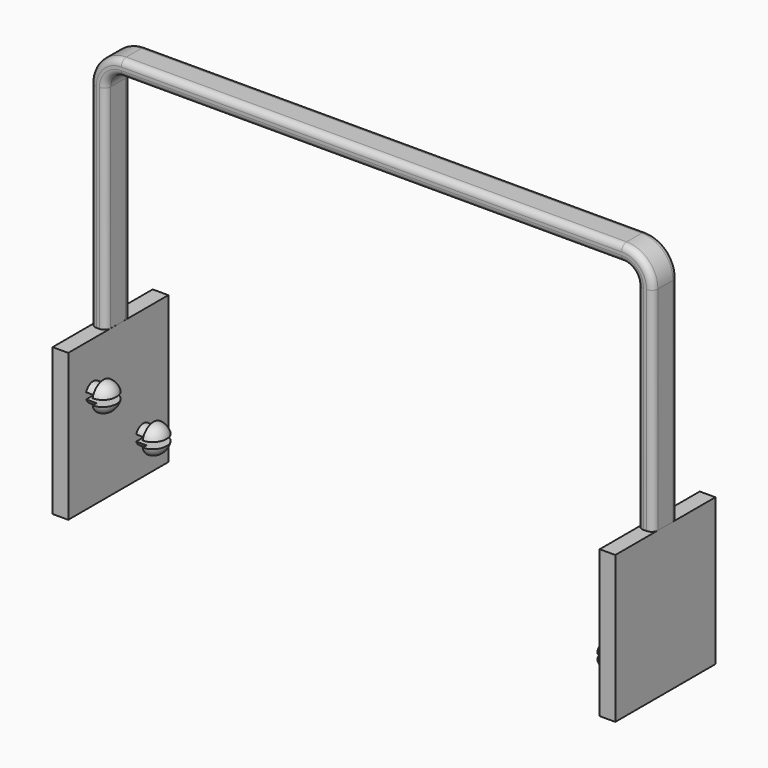
from build123d import *

# Parameters (mm, degrees)
F1_DEPTH  = 10
F2_R      = 2
F3_W      = 5
F3_H      = 40
F4_DEPTH  = 47
F5_R      = 3
F6_DEPTH  = 8.3
F7_R      = 3
F8_DEPTH  = 8.3
F9_R      = 4.5
F10_DEPTH = 4.2
F11_R     = 4.19999
F12_R     = 4.5
F13_DEPTH = 4.2
F14_R     = 4.19999
F16_W     = 169.9655776749
F16_H     = 34.9020669237
F17_DEPTH = 2
F19_W     = 169.9655776749
F19_H     = 34.5512824133
F20_DEPTH = 2


# Not quite as in the source:
# - a fillet or chamfer is up to 0.001 mm smaller than in the source, because OpenCascade refuses the exact size


with BuildPart() as f1:
    # F0 (on Front) → F1 (new body)
    with BuildSketch(Plane.XZ):
        with BuildLine():
            Line((80, 78), (0, 78))
            Line((0, 78), (-80, 78))
            ThreePointArc((-80, 78), (-87.0710678119, 75.0710678119), (-90, 68))
            Line((-90, 68), (-90, 0))
            Line((-90, 0), (-85, 0))
            Line((-85, 0), (-85, 68))
            ThreePointArc((-85, 68), (-83.5355339059, 71.5355339059), (-80, 73))
            Line((-80, 73), (0, 73))
            Line((0, 73), (80, 73))
            ThreePointArc((80, 73), (83.5355339059, 71.5355339059), (85, 68))
            Line((85, 68), (85, 0))
            Line((85, 0), (90, 0))
            Line((90, 0), (90, 68))
            ThreePointArc((90, 68), (87.0710678119, 75.0710678119), (80, 78))
        make_face()
    extrude(amount=F1_DEPTH)

    # F2
    f2_edges = [f1.edges().sort_by_distance(p)[0] for p in [
        (0, -10, 78),
        (0, -10, 73),
        (90, 0, 34),
        (85, 0, 34),
    ]]
    fillet(f2_edges, radius=F2_R)

    # F3 (on face) → F4 (join)
    with BuildSketch(Plane(origin=(0, 0, 0), x_dir=(1, 0, 0), z_dir=(0, 0, -1))):
        with Locations((-87.4827888374, 5)):
            Rectangle(F3_W, F3_H)
        with Locations((87.4827888374, 5)):
            Rectangle(F3_W, F3_H)
    extrude(amount=F4_DEPTH)

    # F5 (on face) → F6 (join)
    with BuildSketch(Plane(origin=(-89.9827888374, 0, 0), x_dir=(0, -1, 0), z_dir=(-1, 0, 0))):
        with Locations((15, -15)):
            Circle(F5_R)
        with Locations((-5, -35)):
            Circle(F5_R)
    extrude(amount=-F6_DEPTH)

    # F7 (on face) → F8 (join)
    with BuildSketch(Plane.YZ.offset(89.9827888374)):
        with Locations((5, -15)):
            Circle(F7_R)
        with Locations((-15, -35)):
            Circle(F7_R)
    extrude(amount=-F8_DEPTH)

    # F9 (on face) → F10 (join)
    with BuildSketch(Plane(origin=(81.6827888374, 0, 0), x_dir=(0, -1, 0), z_dir=(-1, 0, 0))):
        with Locations((-5, -15)):
            Circle(F9_R)
        with Locations((15, -35)):
            Circle(F9_R)
    extrude(amount=F10_DEPTH)

    # F11 (radius 4.2 in the source; OpenCascade refuses exactly that, so slightly less here)
    f11_edges = [f1.edges().sort_by_distance(p)[0] for p in [
        (77.482789, 9.5, -15),
        (77.482789, -10.5, -35),
    ]]
    fillet(f11_edges, radius=F11_R)

    # F12 (on face) → F13 (join)
    with BuildSketch(Plane.YZ.offset(-81.6827888374)):
        with Locations((-15, -15)):
            Circle(F12_R)
        with Locations((5, -35)):
            Circle(F12_R)
    extrude(amount=F13_DEPTH)

    # F14 (radius 4.2 in the source; OpenCascade refuses exactly that, so slightly less here)
    f14_edges = [f1.edges().sort_by_distance(p)[0] for p in [
        (-77.482789, -19.5, -15),
        (-77.482789, 0.5, -35),
    ]]
    fillet(f14_edges, radius=F14_R)

    # F16 (on offset) → F17 (cut)
    with BuildSketch(Plane.XY.offset(-16)):
        with Locations((0, -5.7238894515)):
            Rectangle(F16_W, F16_H)
    extrude(amount=F17_DEPTH, mode=Mode.SUBTRACT)

    # F19 (on offset) → F20 (cut)
    with BuildSketch(Plane.XY.offset(-36)):
        with Locations((0, -5.0480770878)):
            Rectangle(F19_W, F19_H)
    extrude(amount=F20_DEPTH, mode=Mode.SUBTRACT)


solid = f1.part
